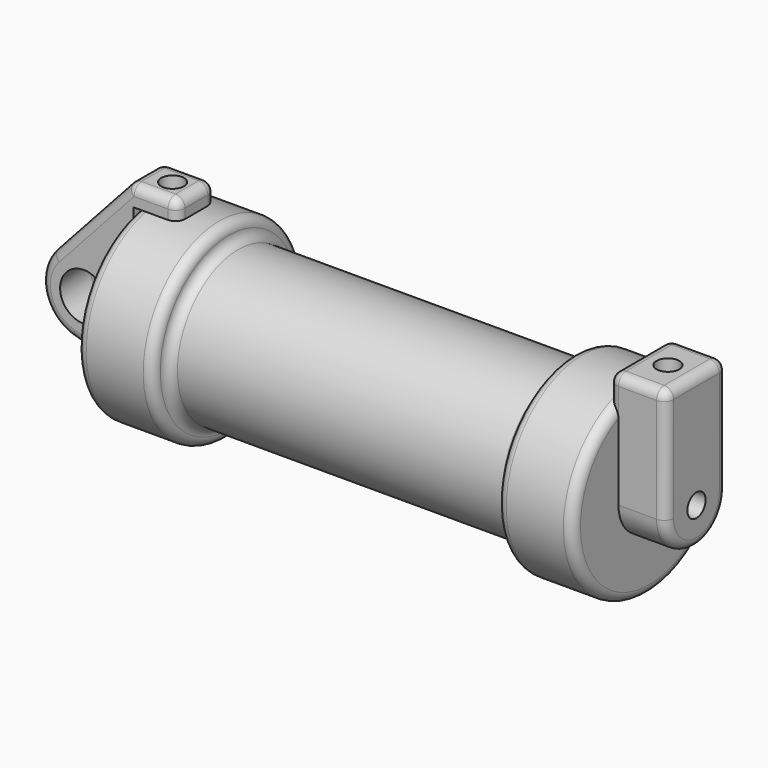
from build123d import *

# Parameters (mm, degrees)
F0_W            = 5.842
F0_H            = 12.7
F0_R            = 3.175
F2_DEPTH        = 3.175
F3_R            = 1.524
F4_DEPTH        = 6.35
F4_DEPTH_BACK   = 1.27
F5_R            = 1.524
F6_DEPTH        = 56.134
F7_R            = 1.524
F8_DEPTH        = 10.414
F9_R            = 1.524
F10_DEPTH       = 17.78
F11_F1_R        = 1.27
F11_F2_R        = 1.2699
F11_2_T1_DEPTH  = 12.7
F11_2_T3_DEPTH  = 9.0167500098
F11_2_T5_DEPTH  = 4.4448500098
F11_2_T7_DEPTH  = 4.5189123252
F11_2_T9_DEPTH  = 14.8459381194
F11_2_T11_DEPTH = 17.7291716486
F11_2_T13_DEPTH = 15.7475000197
F11_2_T15_DEPTH = 3.8102
F11_2_S19_W     = 1.2954
F11_2_S19_H     = 1.2954
F11_2_T20_DEPTH = 1.2954
F11_2_T26_DEPTH = 1.2954
F11_2_S31_W     = 1.2954
F11_2_S31_H     = 1.2954
F11_2_T32_DEPTH = 1.2954
F11_2_T38_DEPTH = 1.2954
F11_2_T42_ANGLE = 116.8111069241
F11_2_T44_ANGLE = 116.8111069241
F11_2_T51_DEPTH = 15.8747500098
F11_2_T55_DEPTH = 12.1915000197
F11_2_T62_DEPTH = 15.8747500098
F11_2_T66_DEPTH = 12.1915000197
F11_3_F1_R      = 1.27
F11_3_F2_R      = 1.27
F11_3_F3_R      = 1.27


# Not quite as in the source:
# - a fillet or chamfer that OpenCascade refuses, or shapes differently, is made with other operations: its cross-section is extruded or revolved along the edge and cut away or added
# - a fillet or chamfer is up to 0.001 mm smaller than in the source, because OpenCascade refuses the exact size


with BuildPart() as f1:
    # F0 (on Front) → F1 (revolve)
    with BuildSketch(Plane.XZ):
        Polygon((5.842, 12.7), (5.842, 0), (66.294, 0), (66.294, 12.7), (56.134, 12.7), (56.134, 10.16), (10.16, 10.16), (10.16, 12.7), align=None)
        with Locations((2.921, 6.35)):
            Rectangle(F0_W, F0_H)
    revolve(axis=Axis((33.147, 0, 0), (-1, 0, 0)))

    # F5 (on face) → F6 (cut, through all)
    with BuildSketch(Plane.YZ.offset(66.294)):
        Circle(F5_R)
    extrude(amount=-F6_DEPTH, mode=Mode.SUBTRACT)

    # F11: fillet of radius 1.27 on 7 edges, made by hand

    # F11_f1
    f11_f1_edges = [f1.edges().sort_by_distance(p)[0] for p in [
        (56.134, 0, -10.16),
        (10.16, 0, -10.16),
    ]]
    fillet(f11_f1_edges, radius=F11_F1_R)

    # F11_f2 (radius 1.27 in the source; OpenCascade refuses exactly that, so slightly less here)
    f11_f2_edges = [f1.edges().sort_by_distance(p)[0] for p in [
        (56.134, 0, -12.7),
        (10.16, 0, -12.7),
        (66.294, 0, -12.7),
        (0, 0, -12.7),
    ]]
    fillet(f11_f2_edges, radius=F11_F2_R)


with BuildPart() as f2:
    # F0 (on Front) → F2 (new body, symmetric)
    with BuildSketch(Plane.XZ):
        with BuildLine():
            Line((-0.9398, 0), (0, 0))
            Line((0, 0), (0, 12.7))
            Line((0, 12.7), (5.842, 12.7))
            Line((5.842, 12.7), (5.842, 15.24))
            Line((5.842, 15.24), (-0.508, 15.24))
            Line((-0.508, 15.24), (-10.8806298187, 3.8475430269))
            ThreePointArc((-10.8806298187, 3.8475430269), (-4.5919612295, 5.3297205562), (-0.9398, 0))
        make_face()
        with BuildLine():
            ThreePointArc((-8.1826630726, -5.5069827884), (-3.1957909266, -4.5493385486), (-0.9398, 0))
            ThreePointArc((-0.9398, 0), (-4.5919612295, 5.3297205562), (-10.8806298187, 3.8475430269))
            ThreePointArc((-10.8806298187, 3.8475430269), (-12.1459778134, -1.5837270034), (-8.1826630726, -5.5069827884))
        make_face()
        with Locations((-6.6548, 0)):
            Circle(F0_R, mode=Mode.SUBTRACT)
        with BuildLine():
            Line((5.842, 0), (0, 0))
            Line((0, 0), (-0.9398, 0))
            ThreePointArc((-0.9398, 0), (-3.1957909266, -4.5493385486), (-8.1826630726, -5.5069827884))
            Line((-8.1826630726, -5.5069827884), (5.842, -9.398))
            Line((5.842, -9.398), (5.842, 0))
        make_face()
    extrude(amount=F2_DEPTH, both=True)

    # F9 (on face) → F10 (cut)
    with BuildSketch(Plane.XY.offset(15.24)):
        with Locations((2.667, 0)):
            Circle(F9_R)
    extrude(amount=-F10_DEPTH, mode=Mode.SUBTRACT)

    # F11#2: fillet of radius 1.27 on 17 edges, made by hand

    # F11_2_s2 → F11_2_t1 (cut)
    with BuildSketch(Plane.XY):
        with BuildLine():
            ThreePointArc((0.0001, 1.9051), (-0.3718743879, 2.8031256121), (-1.2699, 3.1751))
            Line((-1.2699, 3.1751), (-1.2699, 3.2005))
            ThreePointArc((-1.2699, 3.2005), (-0.63495, 3.2004), (0, 3.2004))
            Line((0, 3.2004), (0.0254, 3.175))
            ThreePointArc((0.0254, 3.175), (0.0254, 2.54005), (0.0255, 1.9051))
            Line((0.0255, 1.9051), (0.0001, 1.9051))
        make_face()
    extrude(amount=F11_2_T1_DEPTH, mode=Mode.SUBTRACT)

    # F11_2_s4 → F11_2_t3 (cut)
    with BuildSketch(Plane.YZ):
        with BuildLine():
            ThreePointArc((3.1751, 13.9699), (2.8031256121, 13.0718743879), (1.9051, 12.6999))
            Line((1.9051, 12.6999), (1.9051, 12.6745))
            ThreePointArc((1.9051, 12.6745), (2.54005, 12.6746), (3.175, 12.6746))
            Line((3.175, 12.6746), (3.2004, 12.7))
            ThreePointArc((3.2004, 12.7), (3.2004, 13.33495), (3.2005, 13.9699))
            Line((3.2005, 13.9699), (3.1751, 13.9699))
        make_face()
        with BuildLine():
            ThreePointArc((3.1751, -1.2699), (2.8031256121, -0.3718743879), (1.9051, 0.0001))
            Line((1.9051, 0.0001), (1.9051, 0.0255))
            ThreePointArc((1.9051, 0.0255), (2.54005, 0.0254), (3.175, 0.0254))
            Line((3.175, 0.0254), (3.2004, 0))
            ThreePointArc((3.2004, 0), (3.2004, -0.63495), (3.2005, -1.2699))
            Line((3.2005, -1.2699), (3.1751, -1.2699))
        make_face()
    extrude(amount=F11_2_T3_DEPTH, mode=Mode.SUBTRACT)

    # F11_2_s6 → F11_2_t5 (cut)
    with BuildSketch(Plane.XY.offset(9.5252499902)):
        with BuildLine():
            ThreePointArc((4.5721, 3.1751), (5.4701256121, 2.8031256121), (5.8421, 1.9051))
            Line((5.8421, 1.9051), (5.8675, 1.9051))
            ThreePointArc((5.8675, 1.9051), (5.8674, 2.54005), (5.8674, 3.175))
            Line((5.8674, 3.175), (5.842, 3.2004))
            ThreePointArc((5.842, 3.2004), (5.20705, 3.2004), (4.5721, 3.2005))
            Line((4.5721, 3.2005), (4.5721, 3.1751))
        make_face()
        with BuildLine():
            ThreePointArc((4.5721, -3.1751), (5.4701256121, -2.8031256121), (5.8421, -1.9051))
            Line((5.8421, -1.9051), (5.8675, -1.9051))
            ThreePointArc((5.8675, -1.9051), (5.8674, -2.54005), (5.8674, -3.175))
            Line((5.8674, -3.175), (5.842, -3.2004))
            ThreePointArc((5.842, -3.2004), (5.20705, -3.2004), (4.5721, -3.2005))
            Line((4.5721, -3.2005), (4.5721, -3.1751))
        make_face()
    extrude(amount=F11_2_T5_DEPTH, mode=Mode.SUBTRACT)

    # F11_2_s8 → F11_2_t7 (cut)
    with BuildSketch(Plane.YZ.offset(0.0531876748)):
        with BuildLine():
            ThreePointArc((3.1751, 13.9701), (2.8031256121, 14.8681256121), (1.9051, 15.2401))
            Line((1.9051, 15.2401), (1.9051, 15.2655))
            ThreePointArc((1.9051, 15.2655), (2.54005, 15.2654), (3.175, 15.2654))
            Line((3.175, 15.2654), (3.2004, 15.24))
            ThreePointArc((3.2004, 15.24), (3.2004, 14.60505), (3.2005, 13.9701))
            Line((3.2005, 13.9701), (3.1751, 13.9701))
        make_face()
        with BuildLine():
            ThreePointArc((-3.1751, 13.9701), (-2.8031256121, 14.8681256121), (-1.9051, 15.2401))
            Line((-1.9051, 15.2401), (-1.9051, 15.2655))
            ThreePointArc((-1.9051, 15.2655), (-2.54005, 15.2654), (-3.175, 15.2654))
            Line((-3.175, 15.2654), (-3.2004, 15.24))
            ThreePointArc((-3.2004, 15.24), (-3.2004, 14.60505), (-3.2005, 13.9701))
            Line((-3.2005, 13.9701), (-3.1751, 13.9701))
        make_face()
    extrude(amount=F11_2_T7_DEPTH, mode=Mode.SUBTRACT)

    # F11_2_s10 → F11_2_t9 (cut)
    with BuildSketch(Plane(origin=(6.9785530444, 0, 7.6646777801), x_dir=(0, 1, 0), z_dir=(-0.6732358752, 0, -0.7394277898))):
        with BuildLine():
            ThreePointArc((3.1751, -9.3658440555), (2.8031256121, -10.2638696676), (1.9051, -10.6358440555))
            Line((1.9051, -10.6358440555), (1.9051, -10.6612440555))
            ThreePointArc((1.9051, -10.6612440555), (2.54005, -10.6611440555), (3.175, -10.6611440555))
            Line((3.175, -10.6611440555), (3.2004, -10.6357440555))
            ThreePointArc((3.2004, -10.6357440555), (3.2004, -10.0007940555), (3.2005, -9.3658440555))
            Line((3.2005, -9.3658440555), (3.1751, -9.3658440555))
        make_face()
        with BuildLine():
            ThreePointArc((-3.1751, -9.3658440555), (-2.8031256121, -10.2638696676), (-1.9051, -10.6358440555))
            Line((-1.9051, -10.6358440555), (-1.9051, -10.6612440555))
            ThreePointArc((-1.9051, -10.6612440555), (-2.54005, -10.6611440555), (-3.175, -10.6611440555))
            Line((-3.175, -10.6611440555), (-3.2004, -10.6357440555))
            ThreePointArc((-3.2004, -10.6357440555), (-3.2004, -10.0007940555), (-3.2005, -9.3658440555))
            Line((-3.2005, -9.3658440555), (-3.1751, -9.3658440555))
        make_face()
    extrude(amount=F11_2_T9_DEPTH, mode=Mode.SUBTRACT)

    # F11_2_s12 → F11_2_t11 (cut)
    with BuildSketch(Plane(origin=(-6.179167626, 0, 1.7143547379), x_dir=(0, 1, 0), z_dir=(0.9636015378, 0, -0.2673426199))):
        with BuildLine():
            ThreePointArc((3.1751, -6.2242116667), (2.8031256121, -7.1222372788), (1.9051, -7.4942116667))
            Line((1.9051, -7.4942116667), (1.9051, -7.5196116667))
            ThreePointArc((1.9051, -7.5196116667), (2.54005, -7.5195116667), (3.175, -7.5195116667))
            Line((3.175, -7.5195116667), (3.2004, -7.4941116667))
            ThreePointArc((3.2004, -7.4941116667), (3.2004, -6.8591616667), (3.2005, -6.2242116667))
            Line((3.2005, -6.2242116667), (3.1751, -6.2242116667))
        make_face()
        with BuildLine():
            ThreePointArc((-3.1751, -6.2242116667), (-2.8031256121, -7.1222372788), (-1.9051, -7.4942116667))
            Line((-1.9051, -7.4942116667), (-1.9051, -7.5196116667))
            ThreePointArc((-1.9051, -7.5196116667), (-2.54005, -7.5195116667), (-3.175, -7.5195116667))
            Line((-3.175, -7.5195116667), (-3.2004, -7.4941116667))
            ThreePointArc((-3.2004, -7.4941116667), (-3.2004, -6.8591616667), (-3.2005, -6.2242116667))
            Line((-3.2005, -6.2242116667), (-3.1751, -6.2242116667))
        make_face()
    extrude(amount=F11_2_T11_DEPTH, mode=Mode.SUBTRACT)

    # F11_2_s14 → F11_2_t13 (cut)
    with BuildSketch(Plane.XY.offset(-12.5727500098)):
        with BuildLine():
            ThreePointArc((4.5721, 3.1751), (5.4701256121, 2.8031256121), (5.8421, 1.9051))
            Line((5.8421, 1.9051), (5.8675, 1.9051))
            ThreePointArc((5.8675, 1.9051), (5.8674, 2.54005), (5.8674, 3.175))
            Line((5.8674, 3.175), (5.842, 3.2004))
            ThreePointArc((5.842, 3.2004), (5.20705, 3.2004), (4.5721, 3.2005))
            Line((4.5721, 3.2005), (4.5721, 3.1751))
        make_face()
    extrude(amount=F11_2_T13_DEPTH, mode=Mode.SUBTRACT)

    # F11_2_s16 → F11_2_t15 (cut)
    with BuildSketch(Plane.XZ.offset(-1.9051)):
        with BuildLine():
            ThreePointArc((5.8421, 13.9701), (5.4701256121, 14.8681256121), (4.5721, 15.2401))
            Line((4.5721, 15.2401), (4.5721, 15.2655))
            ThreePointArc((4.5721, 15.2655), (5.20705, 15.2654), (5.842, 15.2654))
            Line((5.842, 15.2654), (5.8674, 15.24))
            ThreePointArc((5.8674, 15.24), (5.8674, 14.60505), (5.8675, 13.9701))
            Line((5.8675, 13.9701), (5.8421, 13.9701))
        make_face()
        with BuildLine():
            ThreePointArc((0.0531876748, 15.2401), (-0.4601532727, 15.1317286289), (-0.8858856182, 14.8251095615))
            Line((-0.8858856182, 14.8251095615), (-0.9046670841, 14.8422097528))
            ThreePointArc((-0.9046670841, 14.8422097528), (-0.7156873036, 15.0496213102), (-0.5267814659, 15.2571001912))
            Line((-0.5267814659, 15.2571001912), (-0.508, 15.2654))
            ThreePointArc((-0.508, 15.2654), (-0.2274061626, 15.2654), (0.0531876748, 15.2655))
            Line((0.0531876748, 15.2655), (0.0531876748, 15.2401))
        make_face()
    extrude(amount=F11_2_T15_DEPTH, mode=Mode.SUBTRACT)


with BuildPart() as f4:
    # F3 (on face) → F4 (new body, two sides)
    with BuildSketch(Plane.YZ.offset(66.294)) as f4_sk:
        with BuildLine():
            ThreePointArc((-5.08, 11.6397422652), (0, 12.7), (5.08, 11.6397422652))
            Line((5.08, 11.6397422652), (5.08, 15.24))
            Line((5.08, 15.24), (-5.08, 15.24))
            Line((-5.08, 15.24), (-5.08, 11.6397422652))
        make_face()
        with BuildLine():
            ThreePointArc((-5.08, 0), (0, 5.08), (5.08, 0))
            Line((5.08, 0), (5.08, 11.6397422652))
            ThreePointArc((5.08, 11.6397422652), (0, 12.7), (-5.08, 11.6397422652))
            Line((-5.08, 11.6397422652), (-5.08, 0))
        make_face()
        with BuildLine():
            ThreePointArc((-5.08, 0), (0, -5.08), (5.08, 0))
            ThreePointArc((5.08, 0), (0, 5.08), (-5.08, 0))
        make_face()
        Circle(F3_R, mode=Mode.SUBTRACT)
    extrude(amount=F4_DEPTH)
    extrude(f4_sk.sketch, amount=-F4_DEPTH_BACK)

    # F7 (on face) → F8 (cut)
    with BuildSketch(Plane.XY.offset(15.24)):
        with Locations((68.834, 0)):
            Circle(F7_R)
    extrude(amount=-F8_DEPTH, mode=Mode.SUBTRACT)

    # F11#3: fillet of radius 1.27 on 10 edges, made by hand

    # F11_3_f1
    f11_3_f1_edges = [f4.edges().sort_by_distance(p)[0] for p in [
        (72.644, 5.08, 7.62),
        (72.644, -5.08, 7.62),
        (72.644, 0, -5.08),
    ]]
    fillet(f11_3_f1_edges, radius=F11_3_F1_R)

    # F11_3_f2
    f11_3_f2_edges = [f4.edges().sort_by_distance(p)[0] for p in [
        (65.024, 5.08, 7.62),
        (65.024, -5.08, 7.62),
        (65.024, 0, -5.08),
    ]]
    fillet(f11_3_f2_edges, radius=F11_3_F2_R)

    # F11_3_f3
    f11_3_f3_edges = [f4.edges().sort_by_distance(p)[0] for p in [
        (72.644, 0, 15.24),
    ]]
    fillet(f11_3_f3_edges, radius=F11_3_F3_R)


with BuildPart() as f11_2_tool18:
    # F11_2_s19 → F11_2_t20 (new body)
    with BuildSketch(Plane.XZ.offset(-1.9051)):
        with Locations((5.2198, 14.6178)):
            Rectangle(F11_2_S19_W, F11_2_S19_H)
    extrude(amount=-F11_2_T20_DEPTH)

    # F11_2_s21 → F11_2_t22 (revolve, cut)
    with BuildSketch(Plane(origin=(4.5721, 1.9051, 13.9701), x_dir=(-0.7071067812, 0, -0.7071067812), z_dir=(0.7071067812, 0, -0.7071067812))):
        with BuildLine():
            ThreePointArc((0, -1.27), (1.27, 0), (0, 1.27))
            Line((0, 1.27), (0, -1.27))
        make_face()
    revolve(axis=Axis((4.5721, 1.9051, 13.9701), (0, 1, 0)), mode=Mode.SUBTRACT)


with BuildPart() as f2_1:
    add(f2.part)

    # F11_2_t17: cut F11_2_tool18
    add(f11_2_tool18.part, mode=Mode.SUBTRACT)


with BuildPart() as f11_2_tool24:
    # F11_2_s25 → F11_2_t26 (new body)
    with BuildSketch(Plane.XZ.offset(-1.9051)):
        Polygon((0.0531876748, 13.9701), (0.0531876748, 15.2655), (-0.5192688288, 15.2655), (-0.9046670841, 14.8422097528), align=None)
    extrude(amount=-F11_2_T26_DEPTH)

    # F11_2_s27 → F11_2_t28 (revolve, cut)
    with BuildSketch(Plane(origin=(0.0531876748, 1.9051, 13.9701), x_dir=(0.4042054705, 0, -0.9146682118), z_dir=(0.9146682118, 0, 0.4042054705))):
        with BuildLine():
            ThreePointArc((0, -1.27), (1.27, 0), (0, 1.27))
            Line((0, 1.27), (0, -1.27))
        make_face()
    revolve(axis=Axis((0.0531876748, 1.9051, 13.9701), (0, 1, 0)), mode=Mode.SUBTRACT)


with BuildPart() as f2_2:
    add(f2_1.part)

    # F11_2_t23: cut F11_2_tool24
    add(f11_2_tool24.part, mode=Mode.SUBTRACT)


with BuildPart() as f11_2_tool30:
    # F11_2_s31 → F11_2_t32 (new body)
    with BuildSketch(Plane.XZ.offset(1.9051)):
        with Locations((5.2198, 14.6178)):
            Rectangle(F11_2_S31_W, F11_2_S31_H)
    extrude(amount=F11_2_T32_DEPTH)

    # F11_2_s33 → F11_2_t34 (revolve, cut)
    with BuildSketch(Plane(origin=(4.5721, -1.9051, 13.9701), x_dir=(-0.7071067812, 0, -0.7071067812), z_dir=(-0.7071067812, 0, 0.7071067812))):
        with BuildLine():
            ThreePointArc((0, -1.27), (1.27, 0), (0, 1.27))
            Line((0, 1.27), (0, -1.27))
        make_face()
    revolve(axis=Axis((4.5721, -1.9051, 13.9701), (0, -1, 0)), mode=Mode.SUBTRACT)


with BuildPart() as f2_3:
    add(f2_2.part)

    # F11_2_t29: cut F11_2_tool30
    add(f11_2_tool30.part, mode=Mode.SUBTRACT)


with BuildPart() as f11_2_tool36:
    # F11_2_s37 → F11_2_t38 (new body)
    with BuildSketch(Plane.XZ.offset(1.9051)):
        Polygon((0.0531876748, 13.9701), (0.0531876748, 15.2655), (-0.5192688288, 15.2655), (-0.9046670841, 14.8422097528), align=None)
    extrude(amount=F11_2_T38_DEPTH)

    # F11_2_s39 → F11_2_t40 (revolve, cut)
    with BuildSketch(Plane(origin=(0.0531876748, -1.9051, 13.9701), x_dir=(0.4042054705, 0, -0.9146682118), z_dir=(-0.9146682118, 0, -0.4042054705))):
        with BuildLine():
            ThreePointArc((0, -1.27), (1.27, 0), (0, 1.27))
            Line((0, 1.27), (0, -1.27))
        make_face()
    revolve(axis=Axis((0.0531876748, -1.9051, 13.9701), (0, -1, 0)), mode=Mode.SUBTRACT)


with BuildPart() as f2_4:
    add(f2_3.part)

    # F11_2_t35: cut F11_2_tool36
    add(f11_2_tool36.part, mode=Mode.SUBTRACT)

    # F11_2_s41 → F11_2_t42 (revolve, cut)
    with BuildSketch(Plane(origin=(-3.0162650989, 0, -3.3128214309), x_dir=(0, 1, 0), z_dir=(0.6732358752, 0, 0.7394277898))):
        with BuildLine():
            ThreePointArc((-3.1751, 9.3658440555), (-2.8031256121, 10.2638696676), (-1.9051, 10.6358440555))
            Line((-1.9051, 10.6358440555), (-1.9051, 10.6612440555))
            ThreePointArc((-1.9051, 10.6612440555), (-2.54005, 10.6611440555), (-3.175, 10.6611440555))
            Line((-3.175, 10.6611440555), (-3.2004, 10.6357440555))
            ThreePointArc((-3.2004, 10.6357440555), (-3.2004, 10.0007940555), (-3.2005, 9.3658440555))
            Line((-3.2005, 9.3658440555), (-3.1751, 9.3658440555))
        make_face()
    revolve(axis=Axis((-6.6548, -3.175, 0), (0, -1, 0)), revolution_arc=F11_2_T42_ANGLE, mode=Mode.SUBTRACT)

    # F11_2_s43 → F11_2_t44 (revolve, cut)
    with BuildSketch(Plane(origin=(-3.0162650989, 0, -3.3128214309), x_dir=(0, 1, 0), z_dir=(0.6732358752, 0, 0.7394277898))):
        with BuildLine():
            ThreePointArc((3.1751, 9.3658440555), (2.8031256121, 10.2638696676), (1.9051, 10.6358440555))
            Line((1.9051, 10.6358440555), (1.9051, 10.6612440555))
            ThreePointArc((1.9051, 10.6612440555), (2.54005, 10.6611440555), (3.175, 10.6611440555))
            Line((3.175, 10.6611440555), (3.2004, 10.6357440555))
            ThreePointArc((3.2004, 10.6357440555), (3.2004, 10.0007940555), (3.2005, 9.3658440555))
            Line((3.2005, 9.3658440555), (3.1751, 9.3658440555))
        make_face()
    revolve(axis=Axis((-6.6548, 3.175, 0), (0, -1, 0)), revolution_arc=F11_2_T44_ANGLE, mode=Mode.SUBTRACT)

    # F11_2_s45 → F11_2_t46 (revolve, cut)
    with BuildSketch(Plane.XY):
        with BuildLine():
            ThreePointArc((-2.2099, 3.1751), (-3.1079256121, 2.8031256121), (-3.4799, 1.9051))
            Line((-3.4799, 1.9051), (-3.5053, 1.9051))
            ThreePointArc((-3.5053, 1.9051), (-3.5052, 2.54005), (-3.5052, 3.175))
            Line((-3.5052, 3.175), (-3.4798, 3.2004))
            ThreePointArc((-3.4798, 3.2004), (-2.84485, 3.2004), (-2.2099, 3.2005))
            Line((-2.2099, 3.2005), (-2.2099, 3.1751))
        make_face()
    revolve(axis=Axis((-6.6548, 3.175, 0), (0, -1, 0)), mode=Mode.SUBTRACT)


with BuildPart() as f11_2_tool49:
    # F11_2_s50 → F11_2_t51 (new body)
    with BuildSketch(Plane.XY.offset(-3.1747500098)):
        with BuildLine():
            ThreePointArc((0.0001, 1.9051), (-0.3718743879, 2.8031256121), (-1.2699, 3.1751))
            Line((-1.2699, 3.1751), (-1.2699, 3.2005))
            ThreePointArc((-1.2699, 3.2005), (-0.63495, 3.2004), (0, 3.2004))
            Line((0, 3.2004), (0.0254, 3.175))
            ThreePointArc((0.0254, 3.175), (0.0254, 2.54005), (0.0255, 1.9051))
            Line((0.0255, 1.9051), (0.0001, 1.9051))
        make_face()
    extrude(amount=F11_2_T51_DEPTH)

    split(bisect_by=Plane.XY, keep=Keep.BOTTOM)


with BuildPart() as f11_2_tool53:
    # F11_2_s54 → F11_2_t55 (new body)
    with BuildSketch(Plane.YZ.offset(9.0167500098)):
        with BuildLine():
            ThreePointArc((3.1751, -1.2699), (2.8031256121, -0.3718743879), (1.9051, 0.0001))
            Line((1.9051, 0.0001), (1.9051, 0.0255))
            ThreePointArc((1.9051, 0.0255), (2.54005, 0.0254), (3.175, 0.0254))
            Line((3.175, 0.0254), (3.2004, 0))
            ThreePointArc((3.2004, 0), (3.2004, -0.63495), (3.2005, -1.2699))
            Line((3.2005, -1.2699), (3.1751, -1.2699))
        make_face()
    extrude(amount=-F11_2_T55_DEPTH)

    split(bisect_by=Plane.YZ, keep=Keep.BOTTOM)


with BuildPart() as f11_2_tool49_1:
    add(f11_2_tool49.part)

    # F11_2_t57: intersect F11_2_tool53
    add(f11_2_tool53.part, mode=Mode.INTERSECT)


with BuildPart() as f2_5:
    add(f2_4.part)

    # F11_2_t47: cut F11_2_tool49
    add(f11_2_tool49_1.part, mode=Mode.SUBTRACT)


with BuildPart() as f11_2_tool60:
    # F11_2_s61 → F11_2_t62 (new body)
    with BuildSketch(Plane.XY):
        with BuildLine():
            ThreePointArc((0.0001, 1.9051), (-0.3718743879, 2.8031256121), (-1.2699, 3.1751))
            Line((-1.2699, 3.1751), (-1.2699, 3.2005))
            ThreePointArc((-1.2699, 3.2005), (-0.63495, 3.2004), (0, 3.2004))
            Line((0, 3.2004), (0.0254, 3.175))
            ThreePointArc((0.0254, 3.175), (0.0254, 2.54005), (0.0255, 1.9051))
            Line((0.0255, 1.9051), (0.0001, 1.9051))
        make_face()
    extrude(amount=F11_2_T62_DEPTH)

    split(bisect_by=Plane.XY.offset(12.7), keep=Keep.TOP)


with BuildPart() as f11_2_tool64:
    # F11_2_s65 → F11_2_t66 (new body)
    with BuildSketch(Plane.YZ.offset(-3.1747500098)):
        with BuildLine():
            ThreePointArc((3.1751, 13.9699), (2.8031256121, 13.0718743879), (1.9051, 12.6999))
            Line((1.9051, 12.6999), (1.9051, 12.6745))
            ThreePointArc((1.9051, 12.6745), (2.54005, 12.6746), (3.175, 12.6746))
            Line((3.175, 12.6746), (3.2004, 12.7))
            ThreePointArc((3.2004, 12.7), (3.2004, 13.33495), (3.2005, 13.9699))
            Line((3.2005, 13.9699), (3.1751, 13.9699))
        make_face()
    extrude(amount=F11_2_T66_DEPTH)

    split(bisect_by=Plane.YZ, keep=Keep.BOTTOM)


with BuildPart() as f11_2_tool60_1:
    add(f11_2_tool60.part)

    # F11_2_t68: intersect F11_2_tool64
    add(f11_2_tool64.part, mode=Mode.INTERSECT)


with BuildPart() as f2_6:
    add(f2_5.part)

    # F11_2_t58: cut F11_2_tool60
    add(f11_2_tool60_1.part, mode=Mode.SUBTRACT)


solid = Compound([f1.part, f4.part, f2_6.part])
